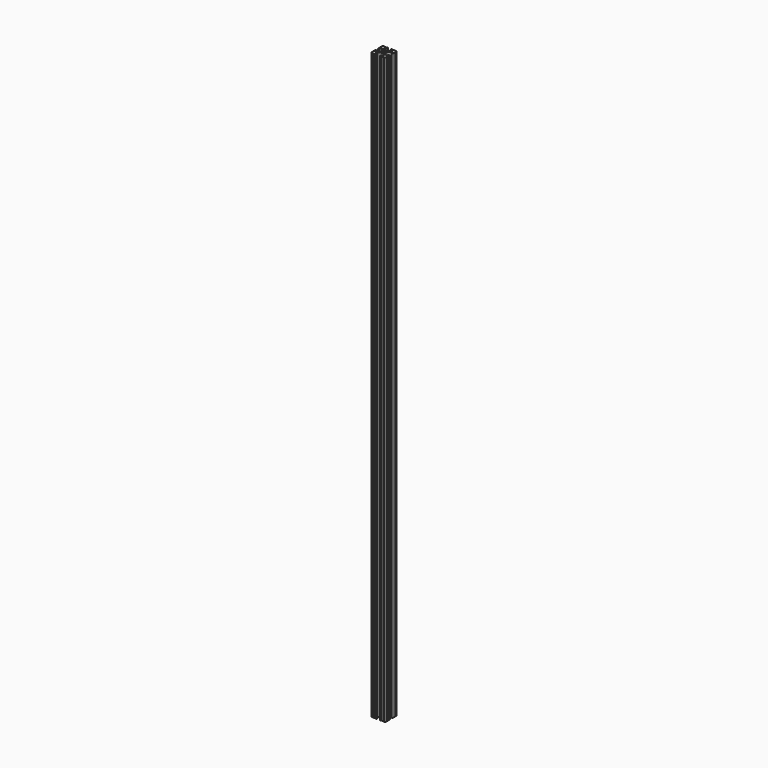
from build123d import *

# Parameters (mm, degrees)
F0_R     = 3.3274
F1_DEPTH = 588.9625
F2_DEPTH = 838.2
F3_DEPTH = 1524


# Not quite as in the source:
# - ends of sketch curves that miss each other by under 0.0002 mm in the source are joined


with BuildPart() as f1:
    # F0 (on Top) → F1 (new body)
    with BuildSketch(Plane.XY):
        with BuildLine():
            ThreePointArc((-10.0228981846, 12.9147496154), (-10.2183621745, 13.207282149), (-10.287, 13.5523478))
            Line((-10.287, 13.5523478), (-10.287, 14.0843))
            ThreePointArc((-10.287, 14.0843), (-10.0228981846, 14.7218981846), (-9.3853, 14.986))
            Line((-9.3853, 14.986), (-5.6176164, 14.986))
            ThreePointArc((-5.6176164, 14.986), (-4.5190437082, 15.4410437082), (-4.064, 16.5396164))
            Line((-4.064, 16.5396164), (-4.064, 17.4963836))
            ThreePointArc((-4.064, 17.4963836), (-4.5190437082, 18.5949562918), (-5.6176164, 19.05))
            Line((-5.6176164, 19.05), (-7.9741776, 19.05))
            ThreePointArc((-7.9741776, 19.05), (-8.7361776, 18.288), (-9.4981776, 19.05))
            Line((-9.4981776, 19.05), (-14.3277082, 19.05))
            ThreePointArc((-14.3277082, 19.05), (-15.0876, 18.2312564), (-15.8474843511, 19.0499994438))
            ThreePointArc((-15.8474843511, 19.0499994438), (-18.1201820503, 18.1202000102), (-19.0500069498, 15.8475171396))
            ThreePointArc((-19.0500069498, 15.8475171396), (-18.2312564, 15.0876254), (-19.0499994438, 14.3277410489))
            Line((-19.0499994438, 14.3277410489), (-19.05, 9.4960948))
            ThreePointArc((-19.05, 9.4960948), (-18.2312564, 8.736203), (-19.0499994438, 7.9763186489))
            Line((-19.0499994438, 7.9763186489), (-19.05, 5.6176164))
            ThreePointArc((-19.05, 5.6176164), (-18.5949562918, 4.5190437082), (-17.4963836, 4.064))
            Line((-17.4963836, 4.064), (-16.5396164, 4.064))
            ThreePointArc((-16.5396164, 4.064), (-15.4410437082, 4.5190437082), (-14.986, 5.6176164))
            Line((-14.986, 5.6176164), (-14.986, 9.3853508))
            ThreePointArc((-14.986, 9.3853508), (-14.7218981846, 10.0229489846), (-14.0843, 10.2870508))
            Line((-14.0843, 10.2870508), (-13.5160512, 10.2870508))
            ThreePointArc((-13.5160512, 10.2870508), (-13.1709772524, 10.2184095379), (-12.8784403156, 10.0229362846))
            Line((-12.8784403156, 10.0229362846), (-8.1475834, 5.2920646))
            ThreePointArc((-8.1475834, 5.2920646), (-7.1179569965, 3.751117767), (-6.7564, 1.933448))
            Line((-6.7564, 1.933448), (-6.7564, -1.933448))
            ThreePointArc((-6.7564, -1.933448), (-7.1179569965, -3.751117767), (-8.1475842107, -5.2920637893))
            Line((-8.1475842107, -5.2920637893), (-12.878435, -10.0229416))
            ThreePointArc((-12.878435, -10.0229416), (-13.1709772524, -10.2184095379), (-13.5160512, -10.2870508))
            Line((-13.5160512, -10.2870508), (-14.0843, -10.2870508))
            ThreePointArc((-14.0843, -10.2870508), (-14.7218981846, -10.0229489846), (-14.986, -9.3853508))
            Line((-14.986, -9.3853508), (-14.986, -5.6176164))
            ThreePointArc((-14.986, -5.6176164), (-15.4410437082, -4.5190437082), (-16.5396164, -4.064))
            Line((-16.5396164, -4.064), (-17.4963836, -4.064))
            ThreePointArc((-17.4963836, -4.064), (-18.5949562918, -4.5190437082), (-19.05, -5.6176164))
            Line((-19.05, -5.6176164), (-19.05, -7.9763112))
            ThreePointArc((-19.05, -7.9763112), (-18.2312564, -8.736203), (-19.0499994438, -9.4960873511))
            Line((-19.0499994438, -9.4960873511), (-19.05, -14.3277336))
            ThreePointArc((-19.05, -14.3277336), (-18.2312564, -15.0876254), (-19.0499994438, -15.8475097511))
            ThreePointArc((-19.0499994438, -15.8475097511), (-18.1201820503, -18.1202000102), (-15.8474917414, -19.0500067288))
            ThreePointArc((-15.8474917414, -19.0500067288), (-15.0876, -18.2312564), (-14.3277156489, -19.0499994438))
            Line((-14.3277156489, -19.0499994438), (-9.4960694, -19.05))
            ThreePointArc((-9.4960694, -19.05), (-8.7361776, -18.2312564), (-7.9762932489, -19.0499994438))
            Line((-7.9762932489, -19.0499994438), (-5.6176164, -19.05))
            ThreePointArc((-5.6176164, -19.05), (-4.5190437082, -18.5949562918), (-4.064, -17.4963836))
            Line((-4.064, -17.4963836), (-4.064, -16.5396164))
            ThreePointArc((-4.064, -16.5396164), (-4.5190437082, -15.4410437082), (-5.6176164, -14.986))
            Line((-5.6176164, -14.986), (-9.3853, -14.986))
            ThreePointArc((-9.3853, -14.986), (-10.0228981846, -14.7218981846), (-10.287, -14.0843))
            Line((-10.287, -14.0843), (-10.287, -13.5523478))
            ThreePointArc((-10.287, -13.5523478), (-10.2183621745, -13.207282149), (-10.0228981846, -12.9147496154))
            Line((-10.0228981846, -12.9147496154), (-5.2521612, -8.144002))
            ThreePointArc((-5.2521612, -8.144002), (-3.7151749705, -7.1170270023), (-1.9021806, -6.7564))
            Line((-1.9021806, -6.7564), (1.9021806, -6.7564))
            ThreePointArc((1.9021806, -6.7564), (3.7151749705, -7.1170270023), (5.2521573829, -8.1440058171))
            Line((5.2521573829, -8.1440058171), (10.0228908, -12.914757))
            ThreePointArc((10.0228908, -12.914757), (10.2183621745, -13.207282149), (10.287, -13.5523478))
            Line((10.287, -13.5523478), (10.287, -14.0843))
            ThreePointArc((10.287, -14.0843), (10.0228981846, -14.7218981846), (9.3853, -14.986))
            Line((9.3853, -14.986), (5.6176164, -14.986))
            ThreePointArc((5.6176164, -14.986), (4.5190437082, -15.4410437082), (4.064, -16.5396164))
            Line((4.064, -16.5396164), (4.064, -17.4963836))
            ThreePointArc((4.064, -17.4963836), (4.5190437082, -18.5949562918), (5.6176164, -19.05))
            Line((5.6176164, -19.05), (7.9762858, -19.05))
            ThreePointArc((7.9762858, -19.05), (8.7361776, -18.2312564), (9.4960619511, -19.0499994438))
            Line((9.4960619511, -19.0499994438), (14.3277082, -19.05))
            ThreePointArc((14.3277082, -19.05), (15.0876, -18.2312564), (15.8474843511, -19.0499994438))
            ThreePointArc((15.8474843511, -19.0499994438), (18.1201820503, -18.1202000102), (19.0500069498, -15.8475171396))
            ThreePointArc((19.0500069498, -15.8475171396), (18.2312564, -15.0876254), (19.0499994438, -14.3277410489))
            Line((19.0499994438, -14.3277410489), (19.05, -9.4960948))
            ThreePointArc((19.05, -9.4960948), (18.2312564, -8.736203), (19.0499994438, -7.9763186489))
            Line((19.0499994438, -7.9763186489), (19.05, -5.6176164))
            ThreePointArc((19.05, -5.6176164), (18.5949562918, -4.5190437082), (17.4963836, -4.064))
            Line((17.4963836, -4.064), (16.5396164, -4.064))
            ThreePointArc((16.5396164, -4.064), (15.4410437082, -4.5190437082), (14.986, -5.6176164))
            Line((14.986, -5.6176164), (14.986, -9.3853508))
            ThreePointArc((14.986, -9.3853508), (14.7218981846, -10.0229489846), (14.0843, -10.2870508))
            Line((14.0843, -10.2870508), (13.5160512, -10.2870508))
            ThreePointArc((13.5160512, -10.2870508), (13.1709772524, -10.2184095379), (12.8784403156, -10.0229362846))
            Line((12.8784403156, -10.0229362846), (8.1475834, -5.2920646))
            ThreePointArc((8.1475834, -5.2920646), (7.1179569965, -3.751117767), (6.7564, -1.933448))
            Line((6.7564, -1.933448), (6.7564, 1.933448))
            ThreePointArc((6.7564, 1.933448), (7.1179569965, 3.751117767), (8.1475842107, 5.2920637893))
            Line((8.1475842107, 5.2920637893), (12.878435, 10.0229416))
            ThreePointArc((12.878435, 10.0229416), (13.1709772524, 10.2184095379), (13.5160512, 10.2870508))
            Line((13.5160512, 10.2870508), (14.0843, 10.2870508))
            ThreePointArc((14.0843, 10.2870508), (14.7218981846, 10.0229489846), (14.986, 9.3853508))
            Line((14.986, 9.3853508), (14.986, 5.6176164))
            ThreePointArc((14.986, 5.6176164), (15.4410437082, 4.5190437082), (16.5396164, 4.064))
            Line((16.5396164, 4.064), (17.4963836, 4.064))
            ThreePointArc((17.4963836, 4.064), (18.5949562918, 4.5190437082), (19.05, 5.6176164))
            Line((19.05, 5.6176164), (19.05, 7.9763112))
            ThreePointArc((19.05, 7.9763112), (18.2312564, 8.736203), (19.0499994438, 9.4960873511))
            Line((19.0499994438, 9.4960873511), (19.05, 14.3277336))
            ThreePointArc((19.05, 14.3277336), (18.2312564, 15.0876254), (19.0499994438, 15.8475097511))
            ThreePointArc((19.0499994438, 15.8475097511), (18.1201820503, 18.1202000102), (15.8474917414, 19.0500067288))
            ThreePointArc((15.8474917414, 19.0500067288), (15.0876, 18.2312564), (14.3277156489, 19.0499994438))
            Line((14.3277156489, 19.0499994438), (9.4981776, 19.05))
            ThreePointArc((9.4981776, 19.05), (8.7361776, 18.288), (7.9741776, 19.05))
            Line((7.9741776, 19.05), (5.6176164, 19.05))
            ThreePointArc((5.6176164, 19.05), (4.5190437082, 18.5949562918), (4.064, 17.4963836))
            Line((4.064, 17.4963836), (4.064, 16.5396164))
            ThreePointArc((4.064, 16.5396164), (4.5190437082, 15.4410437082), (5.6176164, 14.986))
            Line((5.6176164, 14.986), (9.3853, 14.986))
            ThreePointArc((9.3853, 14.986), (10.0228981846, 14.7218981846), (10.287, 14.0843))
            Line((10.287, 14.0843), (10.287, 13.5523478))
            ThreePointArc((10.287, 13.5523478), (10.2183621745, 13.207282149), (10.0228981846, 12.9147496154))
            Line((10.0228981846, 12.9147496154), (5.2521612, 8.144002))
            ThreePointArc((5.2521612, 8.144002), (3.7151749705, 7.1170270023), (1.9021806, 6.7564))
            Line((1.9021806, 6.7564), (-1.9021806, 6.7564))
            ThreePointArc((-1.9021806, 6.7564), (-3.7151749705, 7.1170270023), (-5.2521573829, 8.1440058171))
            Line((-5.2521573829, 8.1440058171), (-10.0228981846, 12.9147496154))
        make_face()
        Circle(F0_R, mode=Mode.SUBTRACT)
    extrude(amount=F1_DEPTH)


with BuildPart() as f2:
    # F0 (on Top) → F2 (new body)
    with BuildSketch(Plane.XY):
        with BuildLine():
            ThreePointArc((-10.0228981846, 12.9147496154), (-10.2183621745, 13.207282149), (-10.287, 13.5523478))
            Line((-10.287, 13.5523478), (-10.287, 14.0843))
            ThreePointArc((-10.287, 14.0843), (-10.0228981846, 14.7218981846), (-9.3853, 14.986))
            Line((-9.3853, 14.986), (-5.6176164, 14.986))
            ThreePointArc((-5.6176164, 14.986), (-4.5190437082, 15.4410437082), (-4.064, 16.5396164))
            Line((-4.064, 16.5396164), (-4.064, 17.4963836))
            ThreePointArc((-4.064, 17.4963836), (-4.5190437082, 18.5949562918), (-5.6176164, 19.05))
            Line((-5.6176164, 19.05), (-7.9741776, 19.05))
            ThreePointArc((-7.9741776, 19.05), (-8.7361776, 18.288), (-9.4981776, 19.05))
            Line((-9.4981776, 19.05), (-14.3277082, 19.05))
            ThreePointArc((-14.3277082, 19.05), (-15.0876, 18.2312564), (-15.8474843511, 19.0499994438))
            ThreePointArc((-15.8474843511, 19.0499994438), (-18.1201820503, 18.1202000102), (-19.0500069498, 15.8475171396))
            ThreePointArc((-19.0500069498, 15.8475171396), (-18.2312564, 15.0876254), (-19.0499994438, 14.3277410489))
            Line((-19.0499994438, 14.3277410489), (-19.05, 9.4960948))
            ThreePointArc((-19.05, 9.4960948), (-18.2312564, 8.736203), (-19.0499994438, 7.9763186489))
            Line((-19.0499994438, 7.9763186489), (-19.05, 5.6176164))
            ThreePointArc((-19.05, 5.6176164), (-18.5949562918, 4.5190437082), (-17.4963836, 4.064))
            Line((-17.4963836, 4.064), (-16.5396164, 4.064))
            ThreePointArc((-16.5396164, 4.064), (-15.4410437082, 4.5190437082), (-14.986, 5.6176164))
            Line((-14.986, 5.6176164), (-14.986, 9.3853508))
            ThreePointArc((-14.986, 9.3853508), (-14.7218981846, 10.0229489846), (-14.0843, 10.2870508))
            Line((-14.0843, 10.2870508), (-13.5160512, 10.2870508))
            ThreePointArc((-13.5160512, 10.2870508), (-13.1709772524, 10.2184095379), (-12.8784403156, 10.0229362846))
            Line((-12.8784403156, 10.0229362846), (-8.1475834, 5.2920646))
            ThreePointArc((-8.1475834, 5.2920646), (-7.1179569965, 3.751117767), (-6.7564, 1.933448))
            Line((-6.7564, 1.933448), (-6.7564, -1.933448))
            ThreePointArc((-6.7564, -1.933448), (-7.1179569965, -3.751117767), (-8.1475842107, -5.2920637893))
            Line((-8.1475842107, -5.2920637893), (-12.878435, -10.0229416))
            ThreePointArc((-12.878435, -10.0229416), (-13.1709772524, -10.2184095379), (-13.5160512, -10.2870508))
            Line((-13.5160512, -10.2870508), (-14.0843, -10.2870508))
            ThreePointArc((-14.0843, -10.2870508), (-14.7218981846, -10.0229489846), (-14.986, -9.3853508))
            Line((-14.986, -9.3853508), (-14.986, -5.6176164))
            ThreePointArc((-14.986, -5.6176164), (-15.4410437082, -4.5190437082), (-16.5396164, -4.064))
            Line((-16.5396164, -4.064), (-17.4963836, -4.064))
            ThreePointArc((-17.4963836, -4.064), (-18.5949562918, -4.5190437082), (-19.05, -5.6176164))
            Line((-19.05, -5.6176164), (-19.05, -7.9763112))
            ThreePointArc((-19.05, -7.9763112), (-18.2312564, -8.736203), (-19.0499994438, -9.4960873511))
            Line((-19.0499994438, -9.4960873511), (-19.05, -14.3277336))
            ThreePointArc((-19.05, -14.3277336), (-18.2312564, -15.0876254), (-19.0499994438, -15.8475097511))
            ThreePointArc((-19.0499994438, -15.8475097511), (-18.1201820503, -18.1202000102), (-15.8474917414, -19.0500067288))
            ThreePointArc((-15.8474917414, -19.0500067288), (-15.0876, -18.2312564), (-14.3277156489, -19.0499994438))
            Line((-14.3277156489, -19.0499994438), (-9.4960694, -19.05))
            ThreePointArc((-9.4960694, -19.05), (-8.7361776, -18.2312564), (-7.9762932489, -19.0499994438))
            Line((-7.9762932489, -19.0499994438), (-5.6176164, -19.05))
            ThreePointArc((-5.6176164, -19.05), (-4.5190437082, -18.5949562918), (-4.064, -17.4963836))
            Line((-4.064, -17.4963836), (-4.064, -16.5396164))
            ThreePointArc((-4.064, -16.5396164), (-4.5190437082, -15.4410437082), (-5.6176164, -14.986))
            Line((-5.6176164, -14.986), (-9.3853, -14.986))
            ThreePointArc((-9.3853, -14.986), (-10.0228981846, -14.7218981846), (-10.287, -14.0843))
            Line((-10.287, -14.0843), (-10.287, -13.5523478))
            ThreePointArc((-10.287, -13.5523478), (-10.2183621745, -13.207282149), (-10.0228981846, -12.9147496154))
            Line((-10.0228981846, -12.9147496154), (-5.2521612, -8.144002))
            ThreePointArc((-5.2521612, -8.144002), (-3.7151749705, -7.1170270023), (-1.9021806, -6.7564))
            Line((-1.9021806, -6.7564), (1.9021806, -6.7564))
            ThreePointArc((1.9021806, -6.7564), (3.7151749705, -7.1170270023), (5.2521573829, -8.1440058171))
            Line((5.2521573829, -8.1440058171), (10.0228908, -12.914757))
            ThreePointArc((10.0228908, -12.914757), (10.2183621745, -13.207282149), (10.287, -13.5523478))
            Line((10.287, -13.5523478), (10.287, -14.0843))
            ThreePointArc((10.287, -14.0843), (10.0228981846, -14.7218981846), (9.3853, -14.986))
            Line((9.3853, -14.986), (5.6176164, -14.986))
            ThreePointArc((5.6176164, -14.986), (4.5190437082, -15.4410437082), (4.064, -16.5396164))
            Line((4.064, -16.5396164), (4.064, -17.4963836))
            ThreePointArc((4.064, -17.4963836), (4.5190437082, -18.5949562918), (5.6176164, -19.05))
            Line((5.6176164, -19.05), (7.9762858, -19.05))
            ThreePointArc((7.9762858, -19.05), (8.7361776, -18.2312564), (9.4960619511, -19.0499994438))
            Line((9.4960619511, -19.0499994438), (14.3277082, -19.05))
            ThreePointArc((14.3277082, -19.05), (15.0876, -18.2312564), (15.8474843511, -19.0499994438))
            ThreePointArc((15.8474843511, -19.0499994438), (18.1201820503, -18.1202000102), (19.0500069498, -15.8475171396))
            ThreePointArc((19.0500069498, -15.8475171396), (18.2312564, -15.0876254), (19.0499994438, -14.3277410489))
            Line((19.0499994438, -14.3277410489), (19.05, -9.4960948))
            ThreePointArc((19.05, -9.4960948), (18.2312564, -8.736203), (19.0499994438, -7.9763186489))
            Line((19.0499994438, -7.9763186489), (19.05, -5.6176164))
            ThreePointArc((19.05, -5.6176164), (18.5949562918, -4.5190437082), (17.4963836, -4.064))
            Line((17.4963836, -4.064), (16.5396164, -4.064))
            ThreePointArc((16.5396164, -4.064), (15.4410437082, -4.5190437082), (14.986, -5.6176164))
            Line((14.986, -5.6176164), (14.986, -9.3853508))
            ThreePointArc((14.986, -9.3853508), (14.7218981846, -10.0229489846), (14.0843, -10.2870508))
            Line((14.0843, -10.2870508), (13.5160512, -10.2870508))
            ThreePointArc((13.5160512, -10.2870508), (13.1709772524, -10.2184095379), (12.8784403156, -10.0229362846))
            Line((12.8784403156, -10.0229362846), (8.1475834, -5.2920646))
            ThreePointArc((8.1475834, -5.2920646), (7.1179569965, -3.751117767), (6.7564, -1.933448))
            Line((6.7564, -1.933448), (6.7564, 1.933448))
            ThreePointArc((6.7564, 1.933448), (7.1179569965, 3.751117767), (8.1475842107, 5.2920637893))
            Line((8.1475842107, 5.2920637893), (12.878435, 10.0229416))
            ThreePointArc((12.878435, 10.0229416), (13.1709772524, 10.2184095379), (13.5160512, 10.2870508))
            Line((13.5160512, 10.2870508), (14.0843, 10.2870508))
            ThreePointArc((14.0843, 10.2870508), (14.7218981846, 10.0229489846), (14.986, 9.3853508))
            Line((14.986, 9.3853508), (14.986, 5.6176164))
            ThreePointArc((14.986, 5.6176164), (15.4410437082, 4.5190437082), (16.5396164, 4.064))
            Line((16.5396164, 4.064), (17.4963836, 4.064))
            ThreePointArc((17.4963836, 4.064), (18.5949562918, 4.5190437082), (19.05, 5.6176164))
            Line((19.05, 5.6176164), (19.05, 7.9763112))
            ThreePointArc((19.05, 7.9763112), (18.2312564, 8.736203), (19.0499994438, 9.4960873511))
            Line((19.0499994438, 9.4960873511), (19.05, 14.3277336))
            ThreePointArc((19.05, 14.3277336), (18.2312564, 15.0876254), (19.0499994438, 15.8475097511))
            ThreePointArc((19.0499994438, 15.8475097511), (18.1201820503, 18.1202000102), (15.8474917414, 19.0500067288))
            ThreePointArc((15.8474917414, 19.0500067288), (15.0876, 18.2312564), (14.3277156489, 19.0499994438))
            Line((14.3277156489, 19.0499994438), (9.4981776, 19.05))
            ThreePointArc((9.4981776, 19.05), (8.7361776, 18.288), (7.9741776, 19.05))
            Line((7.9741776, 19.05), (5.6176164, 19.05))
            ThreePointArc((5.6176164, 19.05), (4.5190437082, 18.5949562918), (4.064, 17.4963836))
            Line((4.064, 17.4963836), (4.064, 16.5396164))
            ThreePointArc((4.064, 16.5396164), (4.5190437082, 15.4410437082), (5.6176164, 14.986))
            Line((5.6176164, 14.986), (9.3853, 14.986))
            ThreePointArc((9.3853, 14.986), (10.0228981846, 14.7218981846), (10.287, 14.0843))
            Line((10.287, 14.0843), (10.287, 13.5523478))
            ThreePointArc((10.287, 13.5523478), (10.2183621745, 13.207282149), (10.0228981846, 12.9147496154))
            Line((10.0228981846, 12.9147496154), (5.2521612, 8.144002))
            ThreePointArc((5.2521612, 8.144002), (3.7151749705, 7.1170270023), (1.9021806, 6.7564))
            Line((1.9021806, 6.7564), (-1.9021806, 6.7564))
            ThreePointArc((-1.9021806, 6.7564), (-3.7151749705, 7.1170270023), (-5.2521573829, 8.1440058171))
            Line((-5.2521573829, 8.1440058171), (-10.0228981846, 12.9147496154))
        make_face()
        Circle(F0_R, mode=Mode.SUBTRACT)
    extrude(amount=F2_DEPTH)


with BuildPart() as f3:
    # F0 (on Top) → F3 (new body)
    with BuildSketch(Plane.XY):
        with BuildLine():
            ThreePointArc((-10.0228981846, 12.9147496154), (-10.2183621745, 13.207282149), (-10.287, 13.5523478))
            Line((-10.287, 13.5523478), (-10.287, 14.0843))
            ThreePointArc((-10.287, 14.0843), (-10.0228981846, 14.7218981846), (-9.3853, 14.986))
            Line((-9.3853, 14.986), (-5.6176164, 14.986))
            ThreePointArc((-5.6176164, 14.986), (-4.5190437082, 15.4410437082), (-4.064, 16.5396164))
            Line((-4.064, 16.5396164), (-4.064, 17.4963836))
            ThreePointArc((-4.064, 17.4963836), (-4.5190437082, 18.5949562918), (-5.6176164, 19.05))
            Line((-5.6176164, 19.05), (-7.9741776, 19.05))
            ThreePointArc((-7.9741776, 19.05), (-8.7361776, 18.288), (-9.4981776, 19.05))
            Line((-9.4981776, 19.05), (-14.3277082, 19.05))
            ThreePointArc((-14.3277082, 19.05), (-15.0876, 18.2312564), (-15.8474843511, 19.0499994438))
            ThreePointArc((-15.8474843511, 19.0499994438), (-18.1201820503, 18.1202000102), (-19.0500069498, 15.8475171396))
            ThreePointArc((-19.0500069498, 15.8475171396), (-18.2312564, 15.0876254), (-19.0499994438, 14.3277410489))
            Line((-19.0499994438, 14.3277410489), (-19.05, 9.4960948))
            ThreePointArc((-19.05, 9.4960948), (-18.2312564, 8.736203), (-19.0499994438, 7.9763186489))
            Line((-19.0499994438, 7.9763186489), (-19.05, 5.6176164))
            ThreePointArc((-19.05, 5.6176164), (-18.5949562918, 4.5190437082), (-17.4963836, 4.064))
            Line((-17.4963836, 4.064), (-16.5396164, 4.064))
            ThreePointArc((-16.5396164, 4.064), (-15.4410437082, 4.5190437082), (-14.986, 5.6176164))
            Line((-14.986, 5.6176164), (-14.986, 9.3853508))
            ThreePointArc((-14.986, 9.3853508), (-14.7218981846, 10.0229489846), (-14.0843, 10.2870508))
            Line((-14.0843, 10.2870508), (-13.5160512, 10.2870508))
            ThreePointArc((-13.5160512, 10.2870508), (-13.1709772524, 10.2184095379), (-12.8784403156, 10.0229362846))
            Line((-12.8784403156, 10.0229362846), (-8.1475834, 5.2920646))
            ThreePointArc((-8.1475834, 5.2920646), (-7.1179569965, 3.751117767), (-6.7564, 1.933448))
            Line((-6.7564, 1.933448), (-6.7564, -1.933448))
            ThreePointArc((-6.7564, -1.933448), (-7.1179569965, -3.751117767), (-8.1475842107, -5.2920637893))
            Line((-8.1475842107, -5.2920637893), (-12.878435, -10.0229416))
            ThreePointArc((-12.878435, -10.0229416), (-13.1709772524, -10.2184095379), (-13.5160512, -10.2870508))
            Line((-13.5160512, -10.2870508), (-14.0843, -10.2870508))
            ThreePointArc((-14.0843, -10.2870508), (-14.7218981846, -10.0229489846), (-14.986, -9.3853508))
            Line((-14.986, -9.3853508), (-14.986, -5.6176164))
            ThreePointArc((-14.986, -5.6176164), (-15.4410437082, -4.5190437082), (-16.5396164, -4.064))
            Line((-16.5396164, -4.064), (-17.4963836, -4.064))
            ThreePointArc((-17.4963836, -4.064), (-18.5949562918, -4.5190437082), (-19.05, -5.6176164))
            Line((-19.05, -5.6176164), (-19.05, -7.9763112))
            ThreePointArc((-19.05, -7.9763112), (-18.2312564, -8.736203), (-19.0499994438, -9.4960873511))
            Line((-19.0499994438, -9.4960873511), (-19.05, -14.3277336))
            ThreePointArc((-19.05, -14.3277336), (-18.2312564, -15.0876254), (-19.0499994438, -15.8475097511))
            ThreePointArc((-19.0499994438, -15.8475097511), (-18.1201820503, -18.1202000102), (-15.8474917414, -19.0500067288))
            ThreePointArc((-15.8474917414, -19.0500067288), (-15.0876, -18.2312564), (-14.3277156489, -19.0499994438))
            Line((-14.3277156489, -19.0499994438), (-9.4960694, -19.05))
            ThreePointArc((-9.4960694, -19.05), (-8.7361776, -18.2312564), (-7.9762932489, -19.0499994438))
            Line((-7.9762932489, -19.0499994438), (-5.6176164, -19.05))
            ThreePointArc((-5.6176164, -19.05), (-4.5190437082, -18.5949562918), (-4.064, -17.4963836))
            Line((-4.064, -17.4963836), (-4.064, -16.5396164))
            ThreePointArc((-4.064, -16.5396164), (-4.5190437082, -15.4410437082), (-5.6176164, -14.986))
            Line((-5.6176164, -14.986), (-9.3853, -14.986))
            ThreePointArc((-9.3853, -14.986), (-10.0228981846, -14.7218981846), (-10.287, -14.0843))
            Line((-10.287, -14.0843), (-10.287, -13.5523478))
            ThreePointArc((-10.287, -13.5523478), (-10.2183621745, -13.207282149), (-10.0228981846, -12.9147496154))
            Line((-10.0228981846, -12.9147496154), (-5.2521612, -8.144002))
            ThreePointArc((-5.2521612, -8.144002), (-3.7151749705, -7.1170270023), (-1.9021806, -6.7564))
            Line((-1.9021806, -6.7564), (1.9021806, -6.7564))
            ThreePointArc((1.9021806, -6.7564), (3.7151749705, -7.1170270023), (5.2521573829, -8.1440058171))
            Line((5.2521573829, -8.1440058171), (10.0228908, -12.914757))
            ThreePointArc((10.0228908, -12.914757), (10.2183621745, -13.207282149), (10.287, -13.5523478))
            Line((10.287, -13.5523478), (10.287, -14.0843))
            ThreePointArc((10.287, -14.0843), (10.0228981846, -14.7218981846), (9.3853, -14.986))
            Line((9.3853, -14.986), (5.6176164, -14.986))
            ThreePointArc((5.6176164, -14.986), (4.5190437082, -15.4410437082), (4.064, -16.5396164))
            Line((4.064, -16.5396164), (4.064, -17.4963836))
            ThreePointArc((4.064, -17.4963836), (4.5190437082, -18.5949562918), (5.6176164, -19.05))
            Line((5.6176164, -19.05), (7.9762858, -19.05))
            ThreePointArc((7.9762858, -19.05), (8.7361776, -18.2312564), (9.4960619511, -19.0499994438))
            Line((9.4960619511, -19.0499994438), (14.3277082, -19.05))
            ThreePointArc((14.3277082, -19.05), (15.0876, -18.2312564), (15.8474843511, -19.0499994438))
            ThreePointArc((15.8474843511, -19.0499994438), (18.1201820503, -18.1202000102), (19.0500069498, -15.8475171396))
            ThreePointArc((19.0500069498, -15.8475171396), (18.2312564, -15.0876254), (19.0499994438, -14.3277410489))
            Line((19.0499994438, -14.3277410489), (19.05, -9.4960948))
            ThreePointArc((19.05, -9.4960948), (18.2312564, -8.736203), (19.0499994438, -7.9763186489))
            Line((19.0499994438, -7.9763186489), (19.05, -5.6176164))
            ThreePointArc((19.05, -5.6176164), (18.5949562918, -4.5190437082), (17.4963836, -4.064))
            Line((17.4963836, -4.064), (16.5396164, -4.064))
            ThreePointArc((16.5396164, -4.064), (15.4410437082, -4.5190437082), (14.986, -5.6176164))
            Line((14.986, -5.6176164), (14.986, -9.3853508))
            ThreePointArc((14.986, -9.3853508), (14.7218981846, -10.0229489846), (14.0843, -10.2870508))
            Line((14.0843, -10.2870508), (13.5160512, -10.2870508))
            ThreePointArc((13.5160512, -10.2870508), (13.1709772524, -10.2184095379), (12.8784403156, -10.0229362846))
            Line((12.8784403156, -10.0229362846), (8.1475834, -5.2920646))
            ThreePointArc((8.1475834, -5.2920646), (7.1179569965, -3.751117767), (6.7564, -1.933448))
            Line((6.7564, -1.933448), (6.7564, 1.933448))
            ThreePointArc((6.7564, 1.933448), (7.1179569965, 3.751117767), (8.1475842107, 5.2920637893))
            Line((8.1475842107, 5.2920637893), (12.878435, 10.0229416))
            ThreePointArc((12.878435, 10.0229416), (13.1709772524, 10.2184095379), (13.5160512, 10.2870508))
            Line((13.5160512, 10.2870508), (14.0843, 10.2870508))
            ThreePointArc((14.0843, 10.2870508), (14.7218981846, 10.0229489846), (14.986, 9.3853508))
            Line((14.986, 9.3853508), (14.986, 5.6176164))
            ThreePointArc((14.986, 5.6176164), (15.4410437082, 4.5190437082), (16.5396164, 4.064))
            Line((16.5396164, 4.064), (17.4963836, 4.064))
            ThreePointArc((17.4963836, 4.064), (18.5949562918, 4.5190437082), (19.05, 5.6176164))
            Line((19.05, 5.6176164), (19.05, 7.9763112))
            ThreePointArc((19.05, 7.9763112), (18.2312564, 8.736203), (19.0499994438, 9.4960873511))
            Line((19.0499994438, 9.4960873511), (19.05, 14.3277336))
            ThreePointArc((19.05, 14.3277336), (18.2312564, 15.0876254), (19.0499994438, 15.8475097511))
            ThreePointArc((19.0499994438, 15.8475097511), (18.1201820503, 18.1202000102), (15.8474917414, 19.0500067288))
            ThreePointArc((15.8474917414, 19.0500067288), (15.0876, 18.2312564), (14.3277156489, 19.0499994438))
            Line((14.3277156489, 19.0499994438), (9.4981776, 19.05))
            ThreePointArc((9.4981776, 19.05), (8.7361776, 18.288), (7.9741776, 19.05))
            Line((7.9741776, 19.05), (5.6176164, 19.05))
            ThreePointArc((5.6176164, 19.05), (4.5190437082, 18.5949562918), (4.064, 17.4963836))
            Line((4.064, 17.4963836), (4.064, 16.5396164))
            ThreePointArc((4.064, 16.5396164), (4.5190437082, 15.4410437082), (5.6176164, 14.986))
            Line((5.6176164, 14.986), (9.3853, 14.986))
            ThreePointArc((9.3853, 14.986), (10.0228981846, 14.7218981846), (10.287, 14.0843))
            Line((10.287, 14.0843), (10.287, 13.5523478))
            ThreePointArc((10.287, 13.5523478), (10.2183621745, 13.207282149), (10.0228981846, 12.9147496154))
            Line((10.0228981846, 12.9147496154), (5.2521612, 8.144002))
            ThreePointArc((5.2521612, 8.144002), (3.7151749705, 7.1170270023), (1.9021806, 6.7564))
            Line((1.9021806, 6.7564), (-1.9021806, 6.7564))
            ThreePointArc((-1.9021806, 6.7564), (-3.7151749705, 7.1170270023), (-5.2521573829, 8.1440058171))
            Line((-5.2521573829, 8.1440058171), (-10.0228981846, 12.9147496154))
        make_face()
        Circle(F0_R, mode=Mode.SUBTRACT)
    extrude(amount=F3_DEPTH)


solid = Compound([f1.part, f2.part, f3.part])
